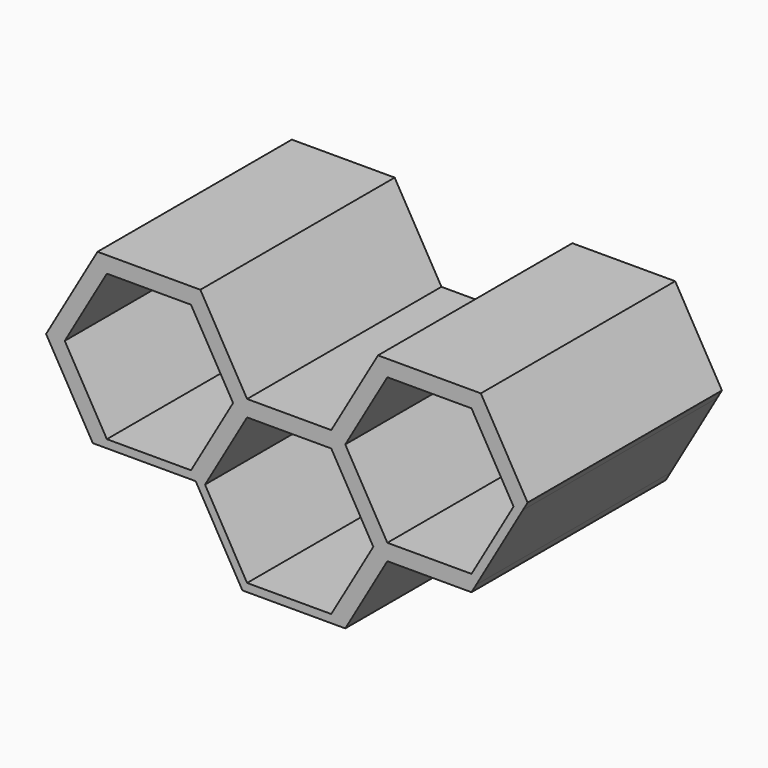
from build123d import *

# Parameters (mm, degrees)
F1_DEPTH = 12.7
F2_DEPTH = 95.25


# Not quite as in the source:
# - a feature names something its author has since deleted; it is built from what else it names


with BuildPart() as f1:
    # F0 (on Front) → F1 (new body)
    with BuildSketch(Plane.XZ):
        Polygon((-169.2561069029, 130.2924993012), (-132.5943648094, 130.2924993012), (-114.2634937626, 162.0424993012), (-132.5943648094, 193.7924993012), (-169.2561069029, 193.7924993012), (-187.5869779497, 162.0424993012), align=None)
        Polygon((-167.4230197982, 133.4674993012), (-183.9208037403, 162.0424993012), (-167.4230197982, 190.6174993012), (-134.427451914, 190.6174993012), (-117.929667972, 162.0424993012), (-134.427451914, 133.4674993012), align=None, mode=Mode.SUBTRACT)
        Polygon((-77.6017516691, 162.0424993012), (-59.2708806223, 130.2924993012), (-27.4963065598, 130.2924993012), (-22.6091385287, 130.2924993012), (-4.278267482, 162.0424993012), (-22.6091385287, 193.7924993012), (-59.2708806223, 193.7924993012), align=None)
        Polygon((-57.4377935176, 133.4674993012), (-73.9355774597, 162.0424993012), (-57.4377935176, 190.6174993012), (-24.4422256334, 190.6174993012), (-7.9444416913, 162.0424993012), (-24.4422256334, 133.4674993012), align=None, mode=Mode.SUBTRACT)
        Polygon((-132.5943648094, 130.2924993012), (-114.2634937626, 98.5424993012), (-77.6017516691, 98.5424993012), (-59.2708806223, 130.2924993012), (-77.6017516691, 162.0424993012), (-114.2634937626, 162.0424993012), align=None)
        Polygon((-112.4304066579, 101.7174993012), (-128.9281906, 130.2924993012), (-112.4304066579, 158.8674993012), (-79.4348387737, 158.8674993012), (-62.9370548316, 130.2924993012), (-79.4348387737, 101.7174993012), align=None, mode=Mode.SUBTRACT)
        Polygon((-57.4377935176, 190.6174993012), (-73.9355774597, 162.0424993012), (-57.4377935176, 133.4674993012), (-24.4422256334, 133.4674993012), (-7.9444416913, 162.0424993012), (-24.4422256334, 190.6174993012), align=None)
        Polygon((-112.4304066579, 158.8674993012), (-128.9281906, 130.2924993012), (-112.4304066579, 101.7174993012), (-79.4348387737, 101.7174993012), (-62.9370548316, 130.2924993012), (-79.4348387737, 158.8674993012), align=None)
        Polygon((-167.4230197982, 190.6174993012), (-183.9208037403, 162.0424993012), (-167.4230197982, 133.4674993012), (-134.427451914, 133.4674993012), (-117.929667972, 162.0424993012), (-134.427451914, 190.6174993012), align=None)
    extrude(amount=F1_DEPTH)

    # F0 (on Front) → F2 (join)
    with BuildSketch(Plane.XZ):
        Polygon((-132.5943648094, 130.2924993012), (-114.2634937626, 98.5424993012), (-77.6017516691, 98.5424993012), (-59.2708806223, 130.2924993012), (-77.6017516691, 162.0424993012), (-114.2634937626, 162.0424993012), align=None)
        Polygon((-112.4304066579, 101.7174993012), (-128.9281906, 130.2924993012), (-112.4304066579, 158.8674993012), (-79.4348387737, 158.8674993012), (-62.9370548316, 130.2924993012), (-79.4348387737, 101.7174993012), align=None, mode=Mode.SUBTRACT)
        Polygon((-59.2708806223, 130.2924993012), (-77.6017516691, 98.5424993012), (-73.9355774597, 98.5424993012), (-57.4377935176, 127.1174993012), (-24.4422256334, 127.1174993012), (-22.6091385287, 130.2924993012), (-27.4963065598, 130.2924993012), align=None)
        Polygon((-169.2561069029, 130.2924993012), (-132.5943648094, 130.2924993012), (-114.2634937626, 162.0424993012), (-132.5943648094, 193.7924993012), (-169.2561069029, 193.7924993012), (-187.5869779497, 162.0424993012), align=None)
        Polygon((-167.4230197982, 133.4674993012), (-183.9208037403, 162.0424993012), (-167.4230197982, 190.6174993012), (-134.427451914, 190.6174993012), (-117.929667972, 162.0424993012), (-134.427451914, 133.4674993012), align=None, mode=Mode.SUBTRACT)
        Polygon((-77.6017516691, 162.0424993012), (-59.2708806223, 130.2924993012), (-27.4963065598, 130.2924993012), (-22.6091385287, 130.2924993012), (-4.278267482, 162.0424993012), (-22.6091385287, 193.7924993012), (-59.2708806223, 193.7924993012), align=None)
        Polygon((-57.4377935176, 133.4674993012), (-73.9355774597, 162.0424993012), (-57.4377935176, 190.6174993012), (-24.4422256334, 190.6174993012), (-7.9444416913, 162.0424993012), (-24.4422256334, 133.4674993012), align=None, mode=Mode.SUBTRACT)
        Polygon((-172.9222811123, 130.2924993012), (-169.2561069029, 130.2924993012), (-187.5869779497, 162.0424993012), (-169.2561069029, 193.7924993012), (-132.5943648094, 193.7924993012), (-114.2634937626, 162.0424993012), (-77.6017516691, 162.0424993012), (-59.2708806223, 193.7924993012), (-22.6091385287, 193.7924993012), (-4.278267482, 162.0424993012), (-2.4451803773, 165.2174993012), (-20.7760514241, 196.9674993012), (-61.103967727, 196.9674993012), (-79.4348387737, 165.2174993012), (-112.4304066579, 165.2174993012), (-130.7612777034, 196.967499299), (-171.0891940088, 196.967499299), (-191.253152159, 162.0424993012), align=None)
    extrude(amount=F2_DEPTH)


solid = f1.part
